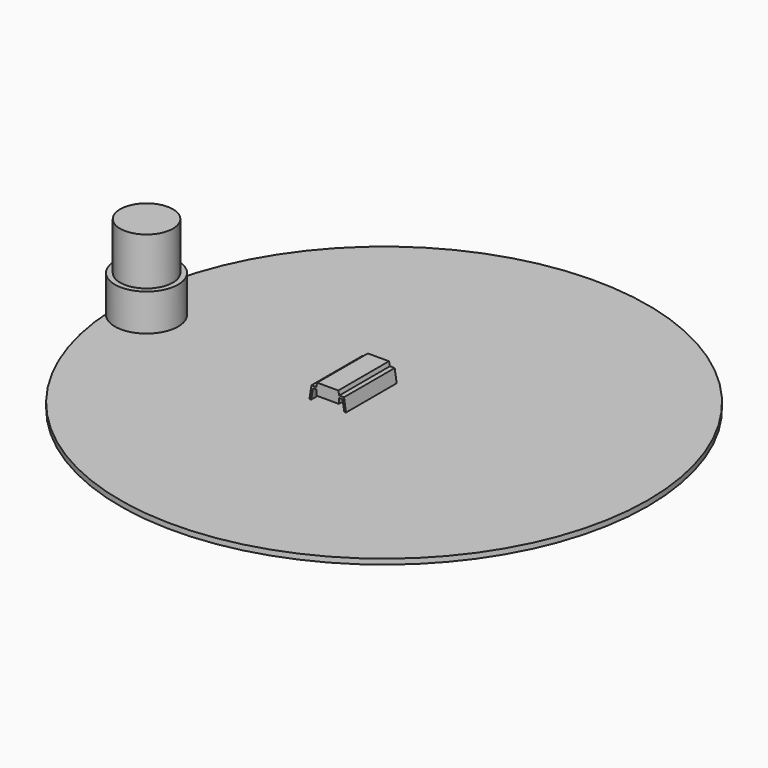
from build123d import *

# Parameters (mm, degrees)
F0_R     = 50
F1_DEPTH = 1
F2_R     = 5
F3_DEPTH = 16
F5_DEPTH = 6
F8_R     = 6
F9_DEPTH = 7


with BuildPart() as f1:
    # F0 (on Top) → F1 (new body)
    with BuildSketch(Plane.XY):
        Circle(F0_R)
    extrude(amount=-F1_DEPTH)


with BuildPart() as f3:
    # F2 (on Top) → F3 (new body)
    with BuildSketch(Plane.XY):
        with Locations((-45, 0)):
            Circle(F2_R)
    extrude(amount=F3_DEPTH)


with BuildPart() as f5:
    # F4 (on Front) → F5 (new body, symmetric)
    with BuildSketch(Plane.XZ):
        Polygon((-8.9535827212, 2.4236521956), (-9.3335827271, 0), (-9.0135823465, 0), (-8.6735826855, 2.0236521658), (-7.9935827688, 2.0236521658), (-7.9935827688, 1), (-5.8735829234, 1), (-5.8735829234, 3.2036522313), (-7.8735829234, 3.2036522313), (-8.0535829888, 2.4236521956), align=None)
    extrude(amount=F5_DEPTH, both=True)

    # F6: F5 across face


with BuildPart() as f5_1:
    add(f5.part)
    add(f5.part.mirror(Plane(origin=(-5.8735829234, 0, 2.1018261156), x_dir=(0, 1, 0), z_dir=(1, 0, 0))))


with BuildPart() as f9:
    # F8 (on Top) → F9 (new body)
    with BuildSketch(Plane.XY):
        with Locations((-45, 0)):
            Circle(F8_R)
    extrude(amount=F9_DEPTH)


solid = Compound([f1.part, f3.part, f5_1.part, f9.part])
